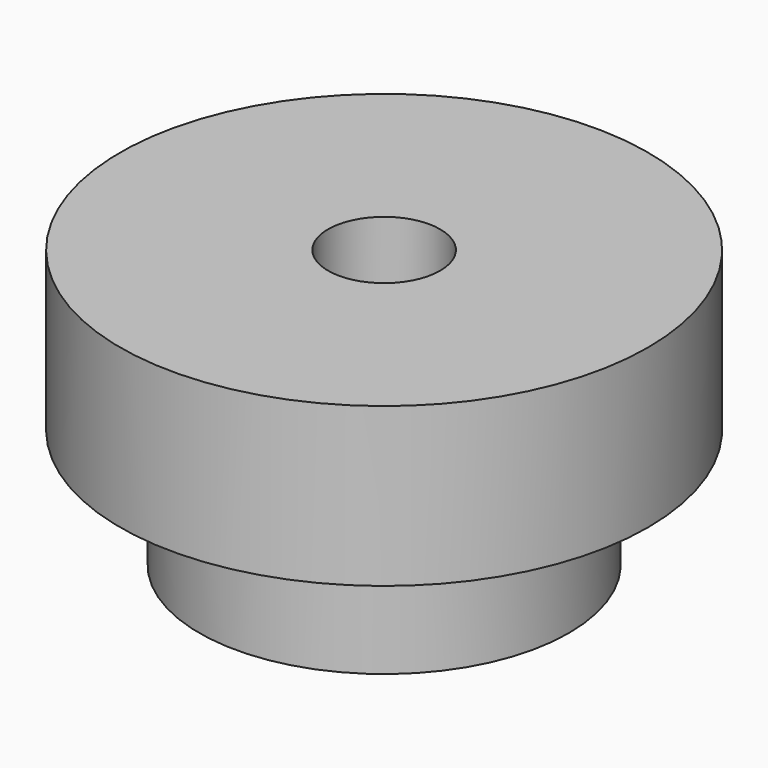
from build123d import *

# Parameters (mm, degrees)
F0_W     = 2
F0_H     = 8
F6_SIZE2 = 1
F6_SIZE  = 2
F7_SIZE2 = 1
F7_SIZE  = 2
F8_R     = 5


with BuildPart() as f1:
    # F0 (on Front) → F1 (revolve)
    with BuildSketch(Plane.XZ):
        with Locations((13, 4)):
            Rectangle(F0_W, F0_H)
    revolve(axis=Axis((0, 0, 16.0184632987), (0, 0, 1)))


with BuildPart() as f3:
    # F2 (on Front) → F3 (revolve)
    with BuildSketch(Plane.XZ):
        Polygon((14.05, 8), (14.05, 1), (20, 1), (20, 13), (4.25, 13), (4.25, -7), (5.95, -7), (5.95, 8), align=None)
    revolve(axis=Axis((0, 0, 8.1785988285), (0, 0, 1)))

    # F6
    f6_edges = [f3.edges().sort_by_distance(p)[0] for p in [
        (-14.05, 0, 1),
    ]]
    chamfer(f6_edges, length=F6_SIZE, length2=F6_SIZE2)

    # F7
    f7_edges = [f3.edges().sort_by_distance(p)[0] for p in [
        (-5.95, 0, -7),
    ]]
    f7_side = f3.faces().sort_by_distance((-5.95, 0, 0.5))[0]
    chamfer(f7_edges, length=F7_SIZE, length2=F7_SIZE2, reference=f7_side)

    # F8
    f8_edges = [f3.edges().sort_by_distance(p)[0] for p in [
        (-14.05, 0, 3),
        (-5.95, 0, -5),
    ]]
    fillet(f8_edges, radius=F8_R)


with BuildPart() as f5:
    # F4 (on Front) → F5 (revolve)
    with BuildSketch(Plane.XZ):
        with BuildLine():
            Line((14, -8), (14, 0))
            Line((14, 0), (12.5, 0))
            Line((12.5, 0), (12.5, -2))
            ThreePointArc((12.5, -2), (10.5, -1.1715728753), (8.5, -2))
            Line((8.5, -2), (8.5, 0))
            Line((8.5, 0), (6, 0))
            Line((6, 0), (6, -8))
            Line((6, -8), (8.5, -8))
            Line((8.5, -8), (8.5, -6))
            ThreePointArc((8.5, -6), (10.5, -6.8284271247), (12.5, -6))
            Line((12.5, -6), (12.5, -8))
            Line((12.5, -8), (14, -8))
        make_face()
    revolve(axis=Axis((0, 0, -10.4025015607), (0, 0, -1)))


solid = Compound([f1.part, f3.part, f5.part])
